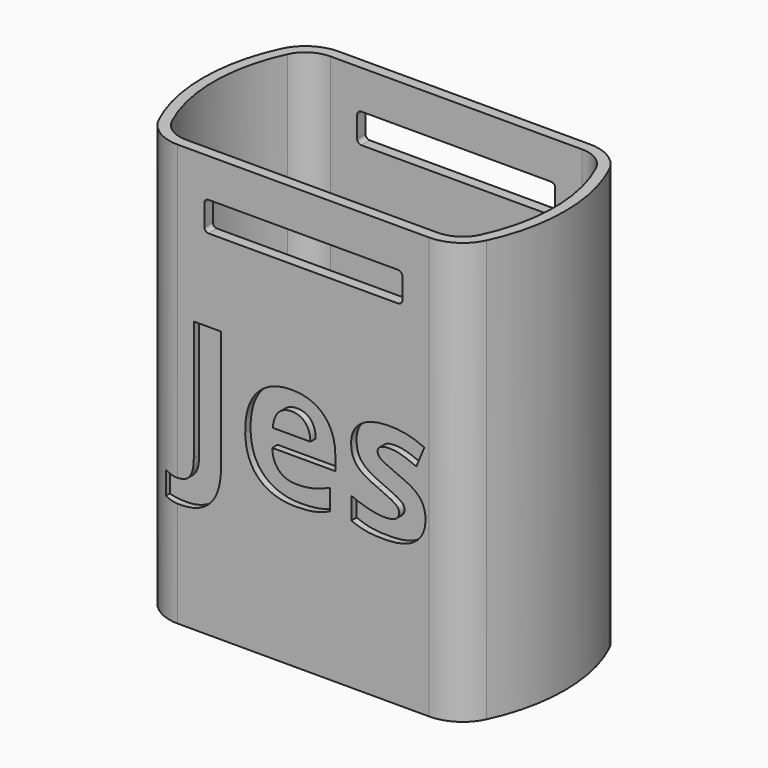
from build123d import *

# Parameters (mm, degrees)
F1_DEPTH     = 127
F2_T         = -3.175
F3_TEXT_SIZE = 54.0321434502
F4_DEPTH     = 2.032
F6_DEPTH     = 60.7124254684


# Not quite as in the source:
# - Text() gives the source's letters only with a copy of the font that has no kerning and outlines rounded to 1/6400 em; it was checked with that copy


with BuildPart() as f1:
    # F0 (on Top) → F1 (new body)
    with BuildSketch(Plane.XY):
        with BuildLine():
            ThreePointArc((-37.849729509, 30.3557127342), (-44.672726301, 28.3672352579), (-49.3591285353, 23.0244867146))
            ThreePointArc((-49.3591285353, 23.0244867146), (-54.4651315819, 0), (-49.3591285353, -23.0244867146))
            ThreePointArc((-49.3591285353, -23.0244867146), (-44.672726301, -28.3672352579), (-37.849729509, -30.3557127342))
            Line((-37.849729509, -30.3557127342), (37.849729509, -30.3557127342))
            ThreePointArc((37.849729509, -30.3557127342), (44.672726301, -28.3672352579), (49.3591285353, -23.0244867146))
            ThreePointArc((49.3591285353, -23.0244867146), (54.4651315819, 0), (49.3591285353, 23.0244867146))
            ThreePointArc((49.3591285353, 23.0244867146), (44.672726301, 28.3672352579), (37.849729509, 30.3557127342))
            Line((37.849729509, 30.3557127342), (-37.849729509, 30.3557127342))
        make_face()
    extrude(amount=F1_DEPTH)

    # F2
    f2_openings = [f1.faces().sort_by_distance(p)[0] for p in [
        (0, 0, 127),
    ]]
    offset(amount=F2_T, openings=f2_openings)

    # F3 (on face) → F4 (cut)
    with BuildSketch(Plane.XZ.offset(30.3557127342)):
        with Locations((-37.849729509, 43.1180345411)):
            Text('Jes', F3_TEXT_SIZE, font='Open Sans', font_style=FontStyle.BOLD, text_align=(TextAlign.LEFT, TextAlign.BOTTOM))
    extrude(amount=-F4_DEPTH, mode=Mode.SUBTRACT)

    # F5 (on face) → F6 (cut, through all)
    with BuildSketch(Plane.XZ.offset(30.3557127342)):
        with BuildLine():
            Line((-28.5537428069, 106.4794361591), (28.5537428069, 106.4794361591))
            ThreePointArc((28.5537428069, 106.4794361591), (29.451768419, 106.851410547), (29.8237428069, 107.7494361591))
            Line((29.8237428069, 107.7494361591), (29.8237428069, 114.1193172741))
            ThreePointArc((29.8237428069, 114.1193172741), (29.451768419, 115.0173428862), (28.5537428069, 115.3893172741))
            Line((28.5537428069, 115.3893172741), (-28.5537428069, 115.3893172741))
            ThreePointArc((-28.5537428069, 115.3893172741), (-29.451768419, 115.0173428862), (-29.8237428069, 114.1193172741))
            Line((-29.8237428069, 114.1193172741), (-29.8237428069, 107.7494361591))
            ThreePointArc((-29.8237428069, 107.7494361591), (-29.451768419, 106.851410547), (-28.5537428069, 106.4794361591))
        make_face()
    extrude(amount=-F6_DEPTH, mode=Mode.SUBTRACT)


solid = f1.part
